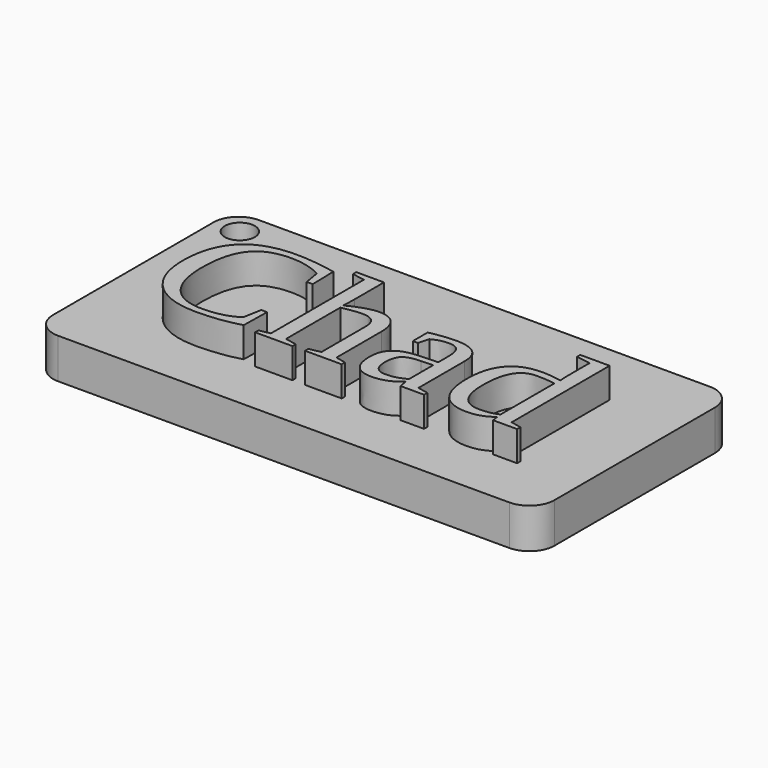
from build123d import *

# Parameters (mm, degrees)
F0_W         = 50
F0_H         = 25
F0_R         = 1.5
F1_DEPTH     = 4
F0_TEXT_SIZE = 18.5078079815
F2_DEPTH     = 7
F3_R         = 2.5


# Not quite as in the source:
# - Text() gives the source's letters only with a copy of the font that has no kerning and outlines rounded to 1/6400 em; it was checked with that copy


with BuildPart() as f1:
    # F0 (on Top) → F1 (new body)
    with BuildSketch(Plane.XY):
        Rectangle(F0_W, F0_H)
        with BuildLine():
            add(Edge.make_bspline(
                [(-8.7304800463, -6.575260014), (-10.7200694043, -7.1449534784), (-13.004626952, -7.1449534784)],
                knots=[0, 0, 0, 1, 1, 1], degree=2))
            add(Edge.make_bspline(
                [(-13.004626952, -7.1449534784), (-15.951417004, -7.1449534784), (-17.5954308849, -5.539979505)],
                knots=[0, 0, 0, 1, 1, 1], degree=2))
            add(Edge.make_bspline(
                [(-17.5954308849, -5.539979505), (-19.2394447658, -3.9350055316), (-19.2394447658, -1.0431605345)],
                knots=[0, 0, 0, 1, 1, 1], degree=2))
            add(Edge.make_bspline(
                [(-19.2394447658, -1.0431605345), (-19.2394447658, 2.0829239074), (-17.6590514748, 3.6878978808)],
                knots=[0, 0, 0, 1, 1, 1], degree=2))
            add(Edge.make_bspline(
                [(-17.6590514748, 3.6878978808), (-16.0786581839, 5.2928718542), (-12.969924812, 5.2928718542)],
                knots=[0, 0, 0, 1, 1, 1], degree=2))
            add(Edge.make_bspline(
                [(-12.969924812, 5.2928718542), (-11.0815500289, 5.2928718542), (-8.9126662811, 4.8301766546)],
                knots=[0, 0, 0, 1, 1, 1], degree=2))
            Line((-8.9126662811, 4.8301766546), (-8.8577212261, 2.1841384823))
            Line((-8.8577212261, 2.1841384823), (-9.4534412955, 2.1841384823))
            Line((-9.4534412955, 2.1841384823), (-9.7252747253, 3.7544103157))
            add(Edge.make_bspline(
                [(-9.7252747253, 3.7544103157), (-10.3585887796, 4.1448093903), (-11.1943319838, 4.3573599976)],
                knots=[0, 0, 0, 1, 1, 1], degree=2))
            add(Edge.make_bspline(
                [(-11.1943319838, 4.3573599976), (-12.030075188, 4.5699106049), (-12.8976286871, 4.5699106049)],
                knots=[0, 0, 0, 1, 1, 1], degree=2))
            add(Edge.make_bspline(
                [(-12.8976286871, 4.5699106049), (-15.2197802198, 4.5699106049), (-16.2854251012, 3.2049597663)],
                knots=[0, 0, 0, 1, 1, 1], degree=2))
            add(Edge.make_bspline(
                [(-16.2854251012, 3.2049597663), (-17.3510699826, 1.8400089276), (-17.3510699826, -1.0258094645)],
                knots=[0, 0, 0, 1, 1, 1], degree=2))
            add(Edge.make_bspline(
                [(-17.3510699826, -1.0258094645), (-17.3510699826, -3.6631721019), (-16.2348178138, -5.055595468)],
                knots=[0, 0, 0, 1, 1, 1], degree=2))
            add(Edge.make_bspline(
                [(-16.2348178138, -5.055595468), (-15.1185656449, -6.4480188341), (-12.987275882, -6.4480188341)],
                knots=[0, 0, 0, 1, 1, 1], degree=2))
            add(Edge.make_bspline(
                [(-12.987275882, -6.4480188341), (-11.957779063, -6.4480188341), (-11.043956044, -6.1993201643)],
                knots=[0, 0, 0, 1, 1, 1], degree=2))
            add(Edge.make_bspline(
                [(-11.043956044, -6.1993201643), (-10.1301330249, -5.9506214946), (-9.5980335454, -5.534195815)],
                knots=[0, 0, 0, 1, 1, 1], degree=2))
            Line((-9.5980335454, -5.534195815), (-9.2625795257, -3.7267926918))
            Line((-9.2625795257, -3.7267926918), (-8.6755349913, -3.7267926918))
            Line((-8.6755349913, -3.7267926918), (-8.7304800463, -6.575260014))
        make_face(mode=Mode.SUBTRACT)
        with BuildLine():
            Line((-4.7079236553, 5.8799163886), (-4.7079236553, 2.2014895523))
            add(Edge.make_bspline(
                [(-4.7079236553, 2.2014895523), (-4.7079236553, 1.2616399282), (-4.7715442452, 0.8452142486)],
                knots=[0, 0, 0, 1, 1, 1], degree=2))
            add(Edge.make_bspline(
                [(-4.7715442452, 0.8452142486), (-4.1208791209, 1.2153704082), (-3.2938114517, 1.487203838)],
                knots=[0, 0, 0, 1, 1, 1], degree=2))
            add(Edge.make_bspline(
                [(-3.2938114517, 1.487203838), (-2.4667437825, 1.7590372677), (-1.8970503181, 1.7590372677)],
                knots=[0, 0, 0, 1, 1, 1], degree=2))
            add(Edge.make_bspline(
                [(-1.8970503181, 1.7590372677), (-0.7952573742, 1.7590372677), (-0.2356853673, 1.1170476783)],
                knots=[0, 0, 0, 1, 1, 1], degree=2))
            add(Edge.make_bspline(
                [(-0.2356853673, 1.1170476783), (0.3238866397, 0.475058089), (0.3238866397, -0.7453004998)],
                knots=[0, 0, 0, 1, 1, 1], degree=2))
            Line((0.3238866397, -0.7453004998), (0.3238866397, -6.3294531892))
            Line((0.3238866397, -6.3294531892), (1.3562753036, -6.555017099))
            Line((1.3562753036, -6.555017099), (1.3562753036, -6.9627672436))
            Line((1.3562753036, -6.9627672436), (-2.3048004627, -6.9627672436))
            Line((-2.3048004627, -6.9627672436), (-2.3048004627, -6.555017099))
            Line((-2.3048004627, -6.555017099), (-1.1740890688, -6.3294531892))
            Line((-1.1740890688, -6.3294531892), (-1.1740890688, -0.8522987647))
            add(Edge.make_bspline(
                [(-1.1740890688, -0.8522987647), (-1.1740890688, 0.7006219988), (-2.6749566223, 0.7006219988)],
                knots=[0, 0, 0, 1, 1, 1], degree=2))
            add(Edge.make_bspline(
                [(-2.6749566223, 0.7006219988), (-3.5251590515, 0.7006219988), (-4.7079236553, 0.437464104)],
                knots=[0, 0, 0, 1, 1, 1], degree=2))
            Line((-4.7079236553, 0.437464104), (-4.7079236553, -6.3294531892))
            Line((-4.7079236553, -6.3294531892), (-3.5598611914, -6.555017099))
            Line((-3.5598611914, -6.555017099), (-3.5598611914, -6.9627672436))
            Line((-3.5598611914, -6.9627672436), (-7.2845575477, -6.9627672436))
            Line((-7.2845575477, -6.9627672436), (-7.2845575477, -6.555017099))
            Line((-7.2845575477, -6.555017099), (-6.2087912088, -6.3294531892))
            Line((-6.2087912088, -6.3294531892), (-6.2087912088, 5.2552778692))
            Line((-6.2087912088, 5.2552778692), (-7.4725274725, 5.472166244))
            Line((-7.4725274725, 5.472166244), (-7.4725274725, 5.8799163886))
            Line((-7.4725274725, 5.8799163886), (-4.7079236553, 5.8799163886))
        make_face(mode=Mode.SUBTRACT)
        with BuildLine():
            add(Edge.make_bspline(
                [(3.2272990168, 1.4062321781), (4.6905725853, 1.7214432827), (5.8010410642, 1.7214432827)],
                knots=[0, 0, 0, 1, 1, 1], degree=2))
            add(Edge.make_bspline(
                [(5.8010410642, 1.7214432827), (7.1920185078, 1.7214432827), (7.8484673222, 1.1517498183)],
                knots=[0, 0, 0, 1, 1, 1], degree=2))
            add(Edge.make_bspline(
                [(7.8484673222, 1.1517498183), (8.5049161365, 0.5820563539), (8.5049161365, -0.5920327149)],
                knots=[0, 0, 0, 1, 1, 1], degree=2))
            Line((8.5049161365, -0.5920327149), (8.5049161365, -6.3294531892))
            Line((8.5049161365, -6.3294531892), (9.5604395604, -6.555017099))
            Line((9.5604395604, -6.555017099), (9.5604395604, -6.9627672436))
            Line((9.5604395604, -6.9627672436), (7.2296124928, -6.9627672436))
            Line((7.2296124928, -6.9627672436), (7.0589936379, -6.1125648144))
            add(Edge.make_bspline(
                [(7.0589936379, -6.1125648144), (6.026604974, -7.1449534784), (4.4274146906, -7.1449534784)],
                knots=[0, 0, 0, 1, 1, 1], degree=2))
            add(Edge.make_bspline(
                [(4.4274146906, -7.1449534784), (2.2498554078, -7.1449534784), (2.2498554078, -4.6116972609)],
                knots=[0, 0, 0, 1, 1, 1], degree=2))
            add(Edge.make_bspline(
                [(2.2498554078, -4.6116972609), (2.2498554078, -3.7643866768), (2.5795257374, -3.2077065148)],
                knots=[0, 0, 0, 1, 1, 1], degree=2))
            add(Edge.make_bspline(
                [(2.5795257374, -3.2077065148), (2.9091960671, -2.6510263529), (3.6321573164, -2.3575040857)],
                knots=[0, 0, 0, 1, 1, 1], degree=2))
            add(Edge.make_bspline(
                [(3.6321573164, -2.3575040857), (4.3551185656, -2.0639818185), (5.7287449393, -2.0379552135)],
                knots=[0, 0, 0, 1, 1, 1], degree=2))
            Line((5.7287449393, -2.0379552135), (7.004048583, -2.0003612285))
            Line((7.004048583, -2.0003612285), (7.004048583, -0.6730043749))
            add(Edge.make_bspline(
                [(7.004048583, -0.6730043749), (7.004048583, 0.2032246593), (6.6830537883, 0.6196503388)],
                knots=[0, 0, 0, 1, 1, 1], degree=2))
            add(Edge.make_bspline(
                [(6.6830537883, 0.6196503388), (6.3620589936, 1.0360760184), (5.6940427993, 1.0360760184)],
                knots=[0, 0, 0, 1, 1, 1], degree=2))
            add(Edge.make_bspline(
                [(5.6940427993, 1.0360760184), (4.7888953152, 1.0360760184), (4.039907461, 0.6109748038)],
                knots=[0, 0, 0, 1, 1, 1], degree=2))
            Line((4.039907461, 0.6109748038), (3.7333718913, -0.4474404651))
            Line((3.7333718913, -0.4474404651), (3.2272990168, -0.4474404651))
            Line((3.2272990168, -0.4474404651), (3.2272990168, 1.4062321781))
        make_face(mode=Mode.SUBTRACT)
        with BuildLine():
            Line((16.4574898785, -6.9627672436), (16.3475997687, -6.3294531892))
            add(Edge.make_bspline(
                [(16.3475997687, -6.3294531892), (15.3267784847, -7.1449534784), (13.961827646, -7.1449534784)],
                knots=[0, 0, 0, 1, 1, 1], degree=2))
            add(Edge.make_bspline(
                [(13.961827646, -7.1449534784), (10.4829381145, -7.1449534784), (10.4829381145, -2.7956186027)],
                knots=[0, 0, 0, 1, 1, 1], degree=2))
            add(Edge.make_bspline(
                [(10.4829381145, -2.7956186027), (10.4829381145, -0.563114265), (11.4690572585, 0.5979615014)],
                knots=[0, 0, 0, 1, 1, 1], degree=2))
            add(Edge.make_bspline(
                [(11.4690572585, 0.5979615014), (12.4551764025, 1.7590372677), (14.3695777906, 1.7590372677)],
                knots=[0, 0, 0, 1, 1, 1], degree=2))
            add(Edge.make_bspline(
                [(14.3695777906, 1.7590372677), (15.3470213997, 1.7590372677), (16.3475997687, 1.5508244279)],
                knots=[0, 0, 0, 1, 1, 1], degree=2))
            add(Edge.make_bspline(
                [(16.3475997687, 1.5508244279), (16.2955465587, 1.8486844626), (16.2955465587, 3.0516919814)],
                knots=[0, 0, 0, 1, 1, 1], degree=2))
            Line((16.2955465587, 3.0516919814), (16.2955465587, 5.2552778692))
            Line((16.2955465587, 5.2552778692), (14.8669751301, 5.472166244))
            Line((14.8669751301, 5.472166244), (14.8669751301, 5.8799163886))
            Line((14.8669751301, 5.8799163886), (17.7935222672, 5.8799163886))
            Line((17.7935222672, 5.8799163886), (17.7935222672, -6.3294531892))
            Line((17.7935222672, -6.3294531892), (18.8432620012, -6.555017099))
            Line((18.8432620012, -6.555017099), (18.8432620012, -6.9627672436))
            Line((18.8432620012, -6.9627672436), (16.4574898785, -6.9627672436))
        make_face(mode=Mode.SUBTRACT)
        with Locations((-22.4327622179, 10.0680400197)):
            Circle(F0_R, mode=Mode.SUBTRACT)
    extrude(amount=F1_DEPTH)

    # F3
    f3_edges = [f1.edges().sort_by_distance(p)[0] for p in [
        (25, 12.5, 2),
        (25, -12.5, 2),
        (-25, 12.5, 2),
        (-25, -12.5, 2),
    ]]
    fillet(f3_edges, radius=F3_R)


with BuildPart() as f1b:
    # F0 (on Top) → F1, piece 2 (new body)
    with BuildSketch(Plane.XY):
        with BuildLine():
            Line((7.004048583, -5.6527614599), (7.004048583, -2.6336752829))
            Line((7.004048583, -2.6336752829), (5.8183921342, -2.6712692679))
            add(Edge.make_bspline(
                [(5.8183921342, -2.6712692679), (4.6096009254, -2.7146469428), (4.1801619433, -3.1397481574)],
                knots=[0, 0, 0, 1, 1, 1], degree=2))
            add(Edge.make_bspline(
                [(4.1801619433, -3.1397481574), (3.7507229612, -3.564849372), (3.7507229612, -4.559644051)],
                knots=[0, 0, 0, 1, 1, 1], degree=2))
            add(Edge.make_bspline(
                [(3.7507229612, -4.559644051), (3.7507229612, -6.1501587994), (5.043377675, -6.1501587994)],
                knots=[0, 0, 0, 1, 1, 1], degree=2))
            add(Edge.make_bspline(
                [(5.043377675, -6.1501587994), (5.6564488143, -6.1501587994), (6.1046847889, -6.009904317)],
                knots=[0, 0, 0, 1, 1, 1], degree=2))
            add(Edge.make_bspline(
                [(6.1046847889, -6.009904317), (6.5529207634, -5.8696498347), (7.004048583, -5.6527614599)],
                knots=[0, 0, 0, 1, 1, 1], degree=2))
        make_face()
    extrude(amount=F1_DEPTH)


with BuildPart() as f1c:
    # F0 (on Top) → F1, piece 3 (new body)
    with BuildSketch(Plane.XY):
        with BuildLine():
            add(Edge.make_bspline(
                [(14.4592249855, 1.0158331034), (12.1110468479, 1.0158331034), (12.1110468479, -2.7956186027)],
                knots=[0, 0, 0, 1, 1, 1], degree=2))
            add(Edge.make_bspline(
                [(12.1110468479, -2.7956186027), (12.1110468479, -4.513374531), (12.6894158473, -5.3577932702)],
                knots=[0, 0, 0, 1, 1, 1], degree=2))
            add(Edge.make_bspline(
                [(12.6894158473, -5.3577932702), (13.2677848467, -6.2022120093), (14.4592249855, -6.2022120093)],
                knots=[0, 0, 0, 1, 1, 1], degree=2))
            add(Edge.make_bspline(
                [(14.4592249855, -6.2022120093), (15.4800462695, -6.2022120093), (16.2955465587, -5.8522987647)],
                knots=[0, 0, 0, 1, 1, 1], degree=2))
            Line((16.2955465587, -5.8522987647), (16.2955465587, 0.8625653186))
            add(Edge.make_bspline(
                [(16.2955465587, 0.8625653186), (15.4916136495, 1.0158331034), (14.4592249855, 1.0158331034)],
                knots=[0, 0, 0, 1, 1, 1], degree=2))
        make_face()
    extrude(amount=F1_DEPTH)


with BuildPart() as f2:
    # F0 (on Top) → F2 (new body)
    with BuildSketch(Plane.XY):
        with Locations((-20, -6.9627672436)):
            Text('Chad', F0_TEXT_SIZE, font='Tinos', text_align=(TextAlign.LEFT, TextAlign.BOTTOM))
    extrude(amount=F2_DEPTH)


solid = Compound([f1.part, f1b.part, f1c.part, f2.part])
